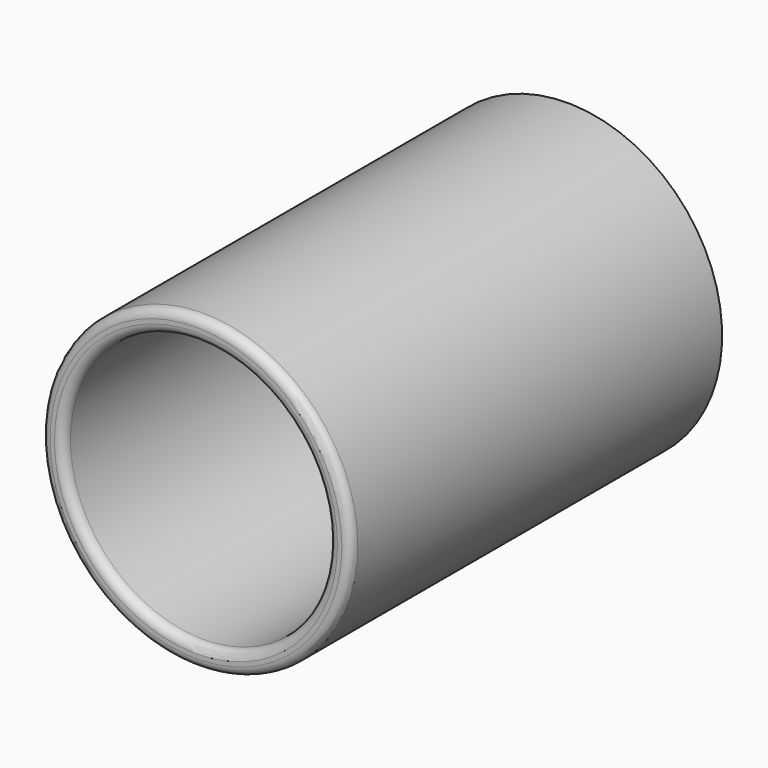
from build123d import *

# Parameters (mm, degrees)
F1_DEPTH    = 123.825
F2_DEPTH    = 25.4
F1_FACE_R   = 44.45
F1_FACE_R_2 = 38.1
F3_DEPTH    = 9.525
F4_R        = 2.54


with BuildPart() as f1:
    # F0 (on Front) → F1 (new body)
    with BuildSketch(Plane.XZ):
        with BuildLine():
            ThreePointArc((44.45, 0), (0, 44.45), (-44.45, 0))
            ThreePointArc((-44.45, 0), (0, -44.45), (44.45, 0))
        make_face()
        with BuildLine():
            ThreePointArc((-38.1, 0), (0, 38.1), (38.1, 0))
            ThreePointArc((38.1, 0), (0, -38.1), (-38.1, 0))
        make_face(mode=Mode.SUBTRACT)
    extrude(amount=F1_DEPTH)

    # F0 (on Front) → F2 (join)
    with BuildSketch(Plane.XZ):
        with BuildLine():
            ThreePointArc((44.45, 0), (0, 44.45), (-44.45, 0))
            ThreePointArc((-44.45, 0), (0, -44.45), (44.45, 0))
        make_face()
        with BuildLine():
            ThreePointArc((-38.1, 0), (0, 38.1), (38.1, 0))
            ThreePointArc((38.1, 0), (0, -38.1), (-38.1, 0))
        make_face(mode=Mode.SUBTRACT)
    extrude(amount=F2_DEPTH)

    # F0 (on Front) + F1_face (on face) → F3 (join)
    with BuildSketch(Plane.XZ):
        with BuildLine():
            ThreePointArc((-38.1, 0), (0, -38.1), (38.1, 0))
            ThreePointArc((38.1, 0), (0, 38.1), (-38.1, 0))
        make_face()
    with BuildSketch(Plane.XZ.offset(123.825)):
        Circle(F1_FACE_R)
        Circle(F1_FACE_R_2, mode=Mode.SUBTRACT)
    extrude(amount=F3_DEPTH)

    # F4
    f4_edges = [f1.edges().sort_by_distance(p)[0] for p in [
        (-44.45, -133.35, 0),
        (-38.1, -133.35, 0),
    ]]
    fillet(f4_edges, radius=F4_R)


solid = f1.part
